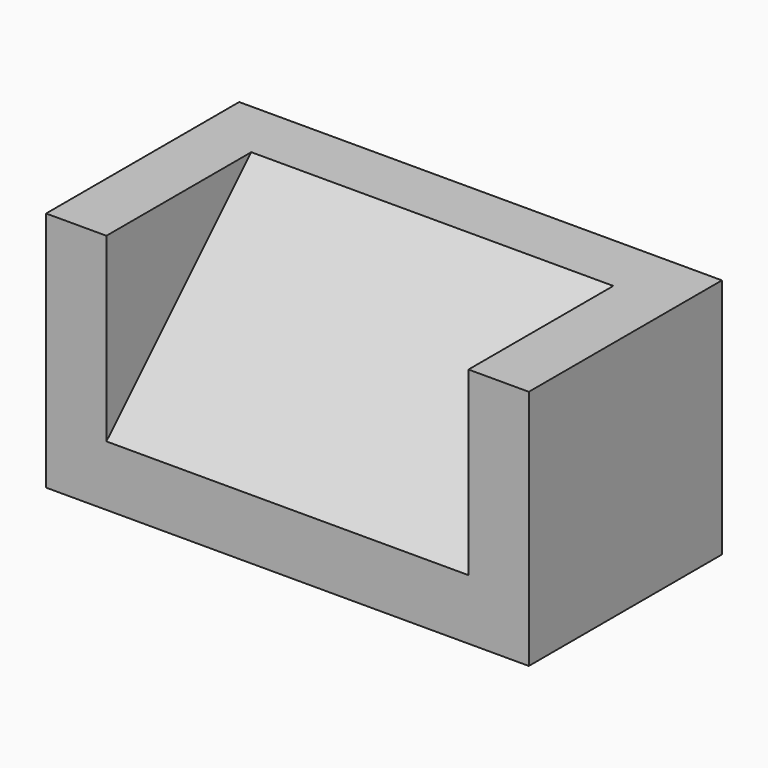
from build123d import *

# Parameters (mm, degrees)
F1_W     = 152.4
F1_H     = 76.2
F2_DEPTH = 101.6
F3_SIZE2 = 76.19999
F3_SIZE  = 76.19999
F5_DEPTH = 101.6


# Not quite as in the source:
# - a fillet or chamfer is up to 0.001 mm smaller than in the source, because OpenCascade refuses the exact size


with BuildPart() as f2:
    # F1 (on face) → F2 (new body)
    with BuildSketch(Plane.XY):
        with Locations((101.6, -63.5)):
            Rectangle(F1_W, F1_H)
    extrude(amount=F2_DEPTH)

    # F3 (size 76.2 and 76.2 in the source; OpenCascade refuses exactly that, so slightly less here)
    f3_edges = [f2.edges().sort_by_distance(p)[0] for p in [
        (101.6, -101.6, 101.6),
    ]]
    chamfer(f3_edges, length=F3_SIZE, length2=F3_SIZE2)

    # F4 (on face) → F5 (join)
    with BuildSketch(Plane.XY):
        Polygon((203.2, 0), (0, 0), (0, -101.6), (25.4, -101.6), (25.4, -25.4), (177.8, -25.4), (177.8, -101.6), (203.2, -101.6), align=None)
    extrude(amount=F5_DEPTH)


solid = f2.part
